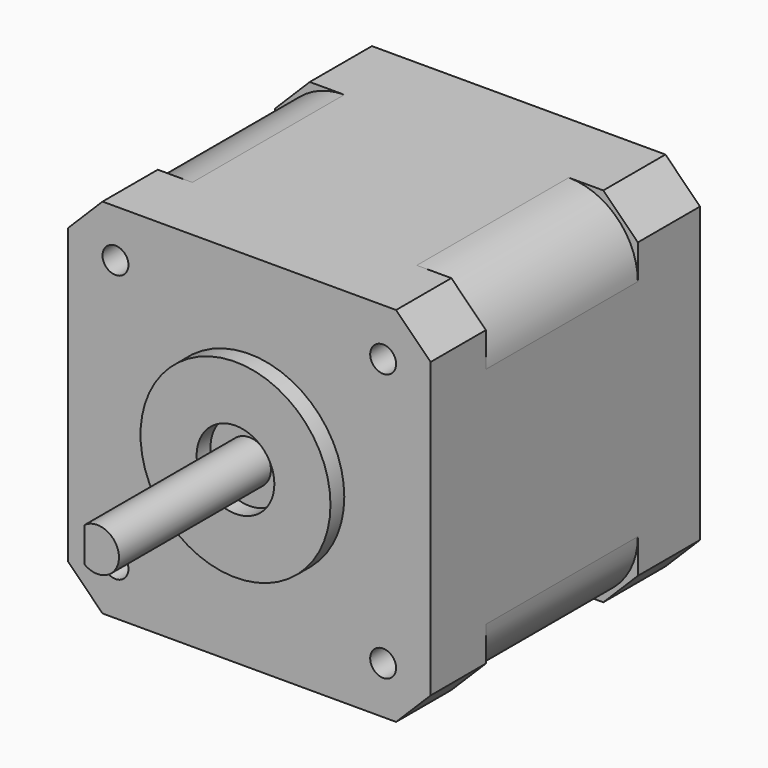
from build123d import *

# Parameters (mm, degrees)
F0_W      = 42
F0_H      = 42
F1_DEPTH  = 8
F3_DEPTH  = 22
F4_W      = 42
F4_H      = 42
F5_DEPTH  = 9
F6_R      = 11
F6_R_2    = 4.5
F7_DEPTH  = 2
F8_R      = 2.5
F9_DEPTH  = 22
F11_DEPTH = 15
F12_R     = 1.5
F13_DEPTH = 4
F14_SIZE  = 4


with BuildPart() as f1:
    # F0 (on Front) → F1 (new body)
    with BuildSketch(Plane.XZ):
        with Locations((21, 21)):
            Rectangle(F0_W, F0_H)
    extrude(amount=F1_DEPTH)

    # F2 (on face) → F3 (join)
    with BuildSketch(Plane(origin=(0, 0, 0), x_dir=(-1, 0, 0), z_dir=(0, 1, 0))):
        with BuildLine():
            Line((0, 8), (0, 21))
            Line((0, 21), (0, 34))
            ThreePointArc((0, 34), (-2.3431457505, 39.6568542495), (-8, 42))
            Line((-8, 42), (-21, 42))
            Line((-21, 42), (-34, 42))
            ThreePointArc((-34, 42), (-39.6568542495, 39.6568542495), (-42, 34))
            Line((-42, 34), (-42, 21))
            Line((-42, 21), (-42, 8))
            ThreePointArc((-42, 8), (-39.6568542495, 2.3431457505), (-34, 0))
            Line((-34, 0), (-21, 0))
            Line((-21, 0), (-8, 0))
            ThreePointArc((-8, 0), (-2.3431457505, 2.3431457505), (0, 8))
        make_face()
    extrude(amount=F3_DEPTH)

    # F4 (on face) → F5 (join)
    with BuildSketch(Plane(origin=(0, 22, 0), x_dir=(-1, 0, 0), z_dir=(0, 1, 0))):
        with Locations((-21, 21)):
            Rectangle(F4_W, F4_H)
    extrude(amount=F5_DEPTH)

    # F6 (on face) → F7 (join)
    with BuildSketch(Plane.XZ.offset(8)):
        with Locations((21, 21)):
            Circle(F6_R)
        with Locations((21, 21)):
            Circle(F6_R_2, mode=Mode.SUBTRACT)
    extrude(amount=F7_DEPTH)

    # F8 (on face) → F9 (join)
    with BuildSketch(Plane.XZ.offset(8)):
        with Locations((21, 21)):
            Circle(F8_R)
    extrude(amount=F9_DEPTH)

    # F10 (on face) → F11 (cut)
    with BuildSketch(Plane.XZ.offset(30)):
        with BuildLine():
            Line((19.5, 19), (19.5, 23))
            ThreePointArc((19.5, 23), (18.7639320225, 22.1180339887), (18.5, 21))
            ThreePointArc((18.5, 21), (18.7639320225, 19.8819660113), (19.5, 19))
        make_face()
    extrude(amount=-F11_DEPTH, mode=Mode.SUBTRACT)

    # F12 (on face) → F13 (cut)
    with BuildSketch(Plane.XZ.offset(8)):
        with Locations((5.5, 5.5)):
            Circle(F12_R)
        with Locations((5.5, 36.5)):
            Circle(F12_R)
        with Locations((36.5, 36.5)):
            Circle(F12_R)
        with Locations((36.5, 5.5)):
            Circle(F12_R)
    extrude(amount=-F13_DEPTH, mode=Mode.SUBTRACT)

    # F14
    f14_edges = [f1.edges().sort_by_distance(p)[0] for p in [
        (0, -4, 42),
        (0, 26.5, 42),
        (42, -4, 42),
        (42, 26.5, 42),
        (42, 26.5, 0),
        (42, -4, 0),
        (0, -4, 0),
        (0, 26.5, 0),
    ]]
    chamfer(f14_edges, length=F14_SIZE)


solid = f1.part
